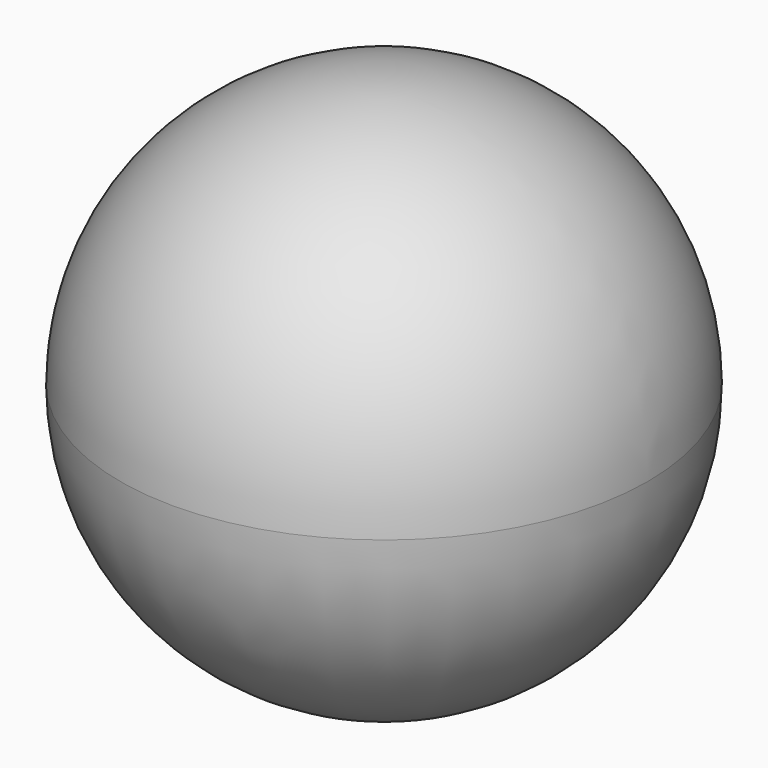
from build123d import *

# Parameters (mm, degrees)
F0_R     = 50.8
F1_DEPTH = 50.8
F2_R     = 50.8
F3_R     = 50.79999


# Not quite as in the source:
# - a fillet or chamfer is up to 0.001 mm smaller than in the source, because OpenCascade refuses the exact size


with BuildPart() as f1:
    # F0 (on Top) → F1 (new body, symmetric)
    with BuildSketch(Plane.XY):
        Circle(F0_R)
    extrude(amount=F1_DEPTH, both=True)

    # F2
    f2_edges = [f1.edges().sort_by_distance(p)[0] for p in [
        (-50.8, 0, 50.8),
    ]]
    fillet(f2_edges, radius=F2_R)

    # F3 (radius 50.8 in the source; OpenCascade refuses exactly that, so slightly less here)
    f3_edges = [f1.edges().sort_by_distance(p)[0] for p in [
        (-50.8, 0, -50.8),
    ]]
    fillet(f3_edges, radius=F3_R)


solid = f1.part
